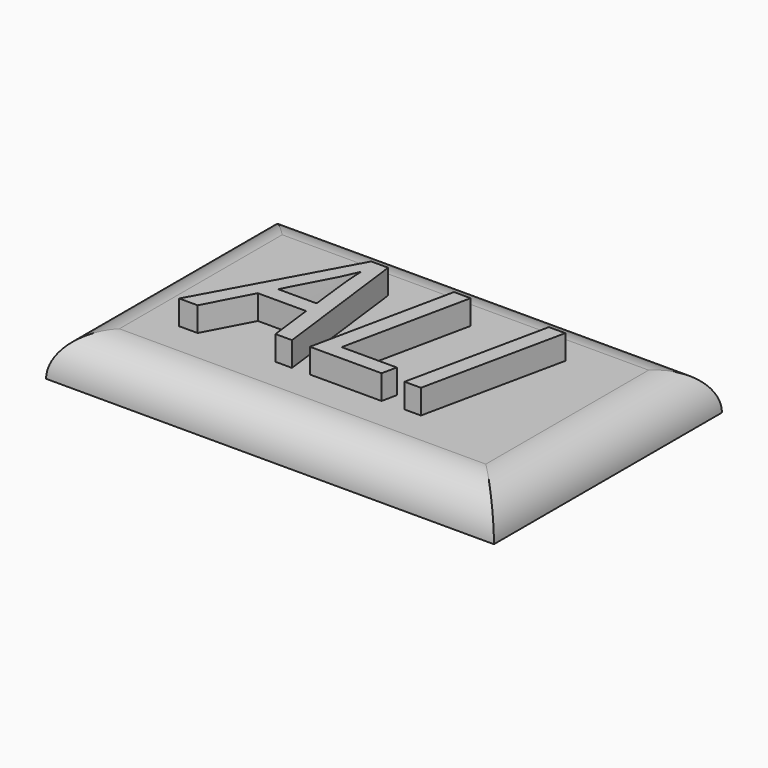
from build123d import *

# Parameters (mm, degrees)
F0_W         = 55
F0_H         = 35
F1_DEPTH     = 5
F2_R         = 4.99999
F3_TEXT_SIZE = 24.52375739
F4_DEPTH     = 3


# Not quite as in the source:
# - a fillet or chamfer is up to 0.001 mm smaller than in the source, because OpenCascade refuses the exact size
# - Text() gives the source's letters only with a copy of the font that has no kerning and outlines rounded to 1/6400 em; it was checked with that copy


with BuildPart() as f1:
    # F0 (on Top) → F1 (new body)
    with BuildSketch(Plane.XY):
        Rectangle(F0_W, F0_H)
    extrude(amount=F1_DEPTH)

    # F2 (radius 5 in the source; OpenCascade refuses exactly that, so slightly less here)
    f2_edges = [f1.edges().sort_by_distance(p)[0] for p in [
        (-27.5, 0, 5),
        (27.5, 0, 5),
        (0, -17.5, 5),
        (0, 17.5, 5),
    ]]
    fillet(f2_edges, radius=F2_R)

    # F3 (on face) → F4 (join)
    with BuildSketch(Plane.XY.offset(5)):
        with Locations((-16.9497672468, -8.499997668)):
            Text('ALI', F3_TEXT_SIZE, font='Open Sans', font_style=FontStyle.ITALIC, text_align=(TextAlign.LEFT, TextAlign.BOTTOM))
    extrude(amount=F4_DEPTH)


solid = f1.part
